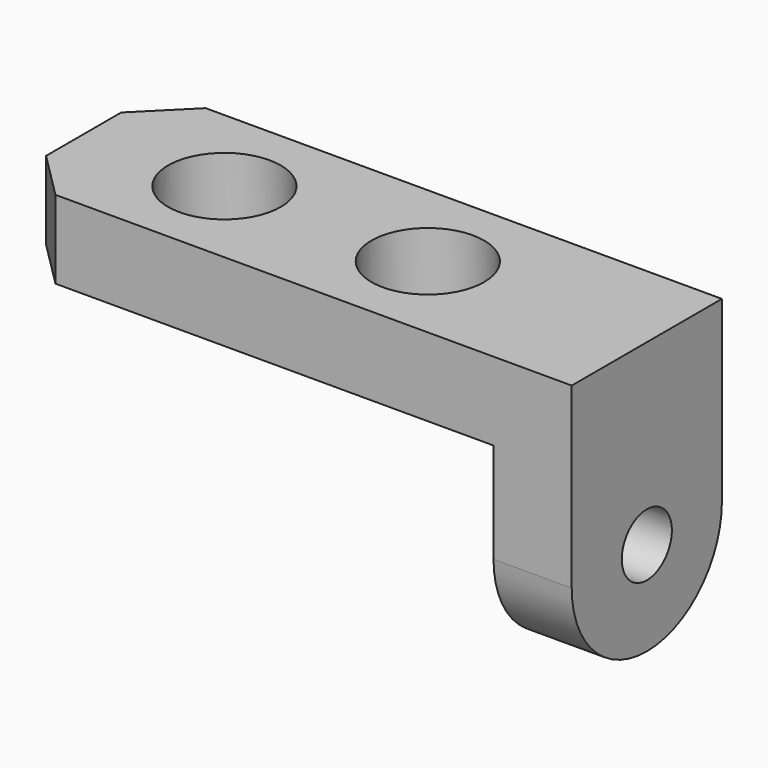
from build123d import *

# Parameters (mm, degrees)
F0_W     = 4572
F0_H     = 1524
F1_DEPTH = 635
F2_W     = 635
F2_H     = 1524
F3_DEPTH = 1574.8
F4_R     = 761.99999
F5_R     = 457.2
F6_DEPTH = 635
F7_R     = 254
F8_DEPTH = 635
F9_SIZE  = 381


# Not quite as in the source:
# - a fillet or chamfer is up to 0.001 mm smaller than in the source, because OpenCascade refuses the exact size


with BuildPart() as f1:
    # F0 (on Top) → F1 (new body)
    with BuildSketch(Plane.XY):
        with Locations((-2286, 762)):
            Rectangle(F0_W, F0_H)
    extrude(amount=F1_DEPTH)

    # F2 (on face) → F3 (join)
    with BuildSketch(Plane(origin=(0, 0, 0), x_dir=(1, 0, 0), z_dir=(0, 0, -1))):
        with Locations((-317.5, -762)):
            Rectangle(F2_W, F2_H)
    extrude(amount=F3_DEPTH)

    # F4 (radius 762 in the source; OpenCascade refuses exactly that, so slightly less here)
    f4_edges = [f1.edges().sort_by_distance(p)[0] for p in [
        (-317.5, 0, -1574.8),
        (-317.5, 1524, -1574.8),
    ]]
    fillet(f4_edges, radius=F4_R)

    # F5 (on face) → F6 (cut)
    with BuildSketch(Plane(origin=(0, 0, 0), x_dir=(1, 0, 0), z_dir=(0, 0, -1))):
        with Locations((-1778, -762)):
            Circle(F5_R)
        with Locations((-3429, -762)):
            Circle(F5_R)
    extrude(amount=-F6_DEPTH, mode=Mode.SUBTRACT)

    # F7 (on face) → F8 (cut, through all)
    with BuildSketch(Plane(origin=(-635, 0, 0), x_dir=(0, -1, 0), z_dir=(-1, 0, 0))):
        with Locations((-762, -812.8)):
            Circle(F7_R)
    extrude(amount=-F8_DEPTH, mode=Mode.SUBTRACT)

    # F9
    f9_edges = [f1.edges().sort_by_distance(p)[0] for p in [
        (-4572, 0, 317.5),
        (-4572, 1524, 317.5),
    ]]
    chamfer(f9_edges, length=F9_SIZE)


solid = f1.part
